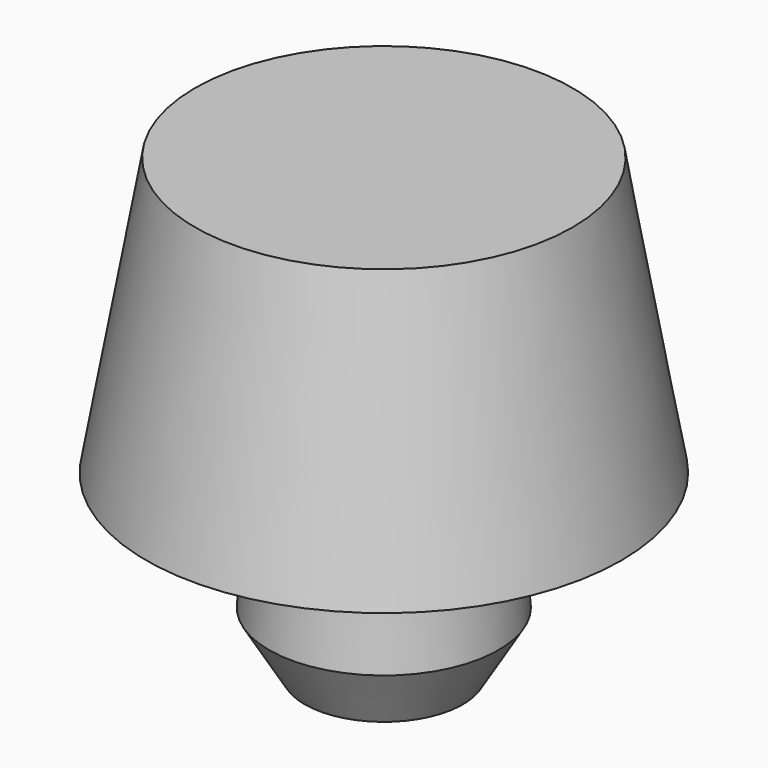
from build123d import *

# Parameters (mm, degrees)
F0_R     = 6
F1_DEPTH = 7
F1_TAPER = 10


# Not quite as in the source:
# - a feature names something its author has since deleted; it is built from what else it names


with BuildPart() as f1:
    # F0 (on Top) → F1 (new body)
    with BuildSketch(Plane.XY):
        Circle(F0_R)
    extrude(amount=F1_DEPTH, taper=F1_TAPER)

    # F2 (on Front) → F3 (revolve)
    with BuildSketch(Plane.XZ):
        Polygon((0, -4.5), (0, 0), (-2.7, 0), (-2.9, -3), (-2, -4.5), align=None)
    revolve(axis=Axis((0, 0, -2.25), (0, 0, 1)))


solid = f1.part
